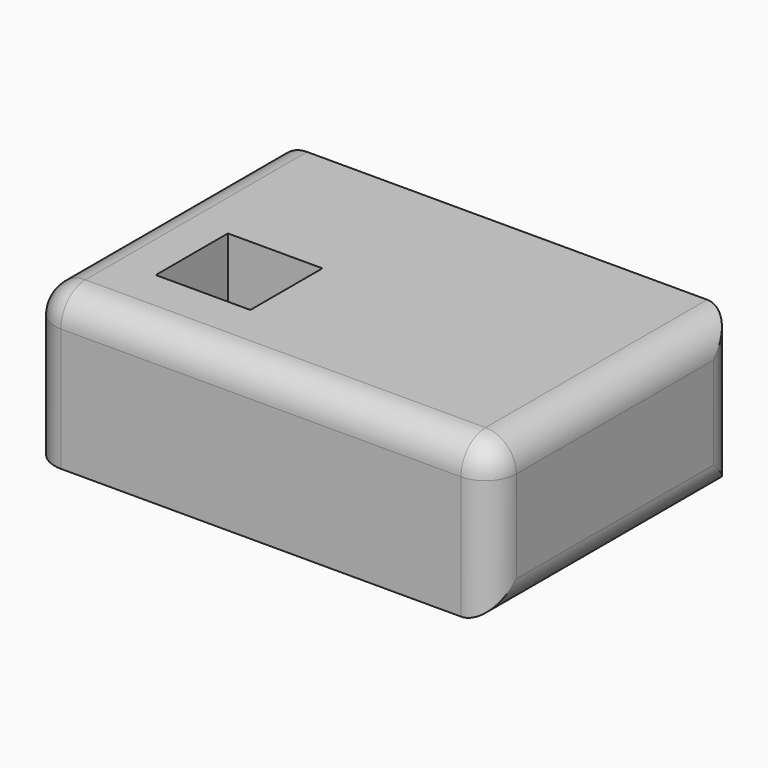
from build123d import *

# Parameters (mm, degrees)
F0_W        = 76.2
F0_H        = 50.8
F1_DEPTH    = 25.4
F2_W        = 15.6074212864
F2_H        = 14.8792807013
F3_DEPTH    = 25.4
F4_R        = 5.08
F5_T        = 2.54
F5_T3_DEPTH = 30.48


# Not quite as in the source:
# - a shell that OpenCascade refuses in one call is made with other operations: the cavity is built on its own and cut out


with BuildPart() as f1:
    # F0 (on Top) → F1 (new body)
    with BuildSketch(Plane.XY):
        with Locations((38.1, 25.4)):
            Rectangle(F0_W, F0_H)
    extrude(amount=F1_DEPTH)

    # F2 (on face) → F3 (cut, through all)
    with BuildSketch(Plane.XY.offset(25.4)):
        with Locations((19.1314755939, 19.2197160795)):
            Rectangle(F2_W, F2_H)
    extrude(amount=-F3_DEPTH, mode=Mode.SUBTRACT)

    # F4
    f4_edges = [f1.edges().sort_by_distance(p)[0] for p in [
        (38.1, 0, 25.4),
        (76.2, 0, 12.7),
        (76.2, 50.8, 12.7),
        (76.2, 25.4, 0),
        (76.2, 25.4, 25.4),
        (0, 0, 12.7),
        (0, 25.4, 25.4),
    ]]
    fillet(f4_edges, radius=F4_R)

    # F5: shell of thickness 2.54, made by hand


with BuildPart() as f5_core1:
    # F5_t2: copy of F1
    add(f1.part)

    # the walls: a layer under each face that stays
    f5_faces = [f5_core1.faces().sort_by_distance(p)[0] for p in [
        (0, 27.94, 10.16),
        (35.56, 50.8, 12.7),
        (1.4878975516, 27.94, 23.9121024484),
        (1.4878975516, 1.4878975516, 10.16),
        (38.1, 27.94, 25.4),
        (74.7121026222, 49.3121022747, 12.7),
        (1.4878975516, 2.54, 22.86),
        (38.1, 0, 10.16),
        (74.7121025744, 25.4, 1.4878976776),
        (11.3277649507, 19.2197160795, 12.7),
        (19.1314755939, 11.7800757289, 12.7),
        (26.9351862371, 19.2197160795, 12.7),
        (19.1314755939, 26.6593564302, 12.7),
        (74.7121026222, 27.94, 23.9121022747),
        (38.1, 1.4878975516, 23.9121024484),
        (76.2, 25.4, 12.7),
        (74.7121024484, 1.4878975516, 10.16),
        (74.7121024484, 2.54, 22.86),
    ]]
    thicken(f5_faces, amount=-F5_T, mode=Mode.SUBTRACT)

    # F5_s4 → F5_t3 (cut)
    with BuildSketch(Plane.XY.offset(-2.54)):
        Polygon((11.3531649507, 26.6339564302), (8.7877649507, 26.6593564302), (8.7877649507, 29.1993564302), (11.3277649507, 29.1993564302), align=None)
        Polygon((11.3531649507, 11.8054757289), (8.7877649507, 11.7800757289), (8.7877649507, 9.2400757289), (11.3277649507, 9.2400757289), align=None)
        Polygon((26.9097862371, 11.8054757289), (26.9351862371, 9.2400757289), (29.4751862371, 9.2400757289), (29.4751862371, 11.7800757289), align=None)
        Polygon((26.9097862371, 26.6339564302), (29.4751862371, 26.6593564302), (29.4751862371, 29.1993564302), (26.9351862371, 29.1993564302), align=None)
    extrude(amount=F5_T3_DEPTH, mode=Mode.SUBTRACT)


with BuildPart() as f1_1:
    add(f1.part)

    # what is left inside the walls is the cavity
    f5_cavity = [f5_core1.part.solids().sort_by_distance(p)[0] for p in [
        (36.83, 17.78, 0.0254),
    ]]
    add(f5_cavity, mode=Mode.SUBTRACT)


solid = f1_1.part
